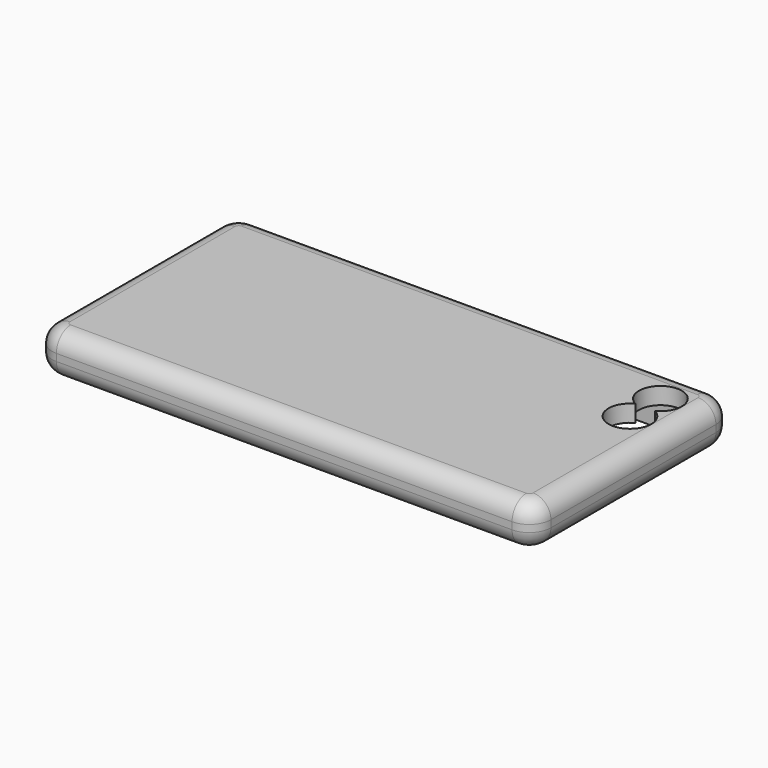
from build123d import *

# Parameters (mm, degrees)
F0_W         = 142.24
F0_H         = 71.12
F1_DEPTH     = 12.192
F3_T         = -4.826
F4_D         = 12.192
F5_R         = 6.1468
F6_T1_DEPTH  = 129.9464
F6_T3_DEPTH  = 58.8264
F6_T6_ANGLE  = 90
F6_T8_ANGLE  = 90
F6_T10_ANGLE = 90
F6_T12_ANGLE = 90
F7_R         = 5.08


# Not quite as in the source:
# - a fillet or chamfer that OpenCascade refuses, or shapes differently, is made with other operations: its cross-section is extruded or revolved along the edge and cut away or added
# - a feature names something its author has since deleted; it is built from what else it names


with BuildPart() as f1:
    # F0 (on Top) → F1 (new body)
    with BuildSketch(Plane.XY):
        Rectangle(F0_W, F0_H)
    extrude(amount=F1_DEPTH)

    # F3
    f3_openings = [f1.faces().sort_by_distance(p)[0] for p in [
        (0, 0, 0),
    ]]
    offset(amount=F3_T, openings=f3_openings)

    # F4 (through all)
    with Locations(Plane(origin=(0, 0, 0), x_dir=(1, 0, 0), z_dir=(0, 0, -1))):
        with Locations((59.7701932977, -12.9658412188), (59.7701932977, -23.8187816803)):
            Hole(F4_D / 2)

    # F5
    f5_edges = [f1.edges().sort_by_distance(p)[0] for p in [
        (66.294, -30.734, 3.683),
        (66.294, 30.734, 3.683),
        (-66.294, 30.734, 3.683),
        (-66.294, -30.734, 3.683),
        (-71.12, 35.56, 6.096),
        (-71.12, -35.56, 6.096),
        (71.12, -35.56, 6.096),
        (71.12, 35.56, 6.096),
    ]]
    fillet(f5_edges, radius=F5_R)

    # F6: fillet of radius 5.08 on 1 edges, made by hand

    # F6_s2 → F6_t1 (cut)
    with BuildSketch(Plane.YZ.offset(-64.9732)):
        with BuildLine():
            ThreePointArc((30.48, 0), (34.0721024484, 1.4878975516), (35.56, 5.08))
            Line((35.56, 5.08), (35.56, 0))
            Line((35.56, 0), (30.48, 0))
        make_face()
        with BuildLine():
            ThreePointArc((-35.56, 5.08), (-34.0721024484, 1.4878975516), (-30.48, 0))
            Line((-30.48, 0), (-35.56, 0))
            Line((-35.56, 0), (-35.56, 5.08))
        make_face()
    extrude(amount=F6_T1_DEPTH, mode=Mode.SUBTRACT)

    # F6_s4 → F6_t3 (cut)
    with BuildSketch(Plane.XZ.offset(-29.4132)):
        with BuildLine():
            ThreePointArc((-66.04, 0), (-69.6321024484, 1.4878975516), (-71.12, 5.08))
            Line((-71.12, 5.08), (-71.12, 0))
            Line((-71.12, 0), (-66.04, 0))
        make_face()
        with BuildLine():
            ThreePointArc((66.04, 0), (69.6321024484, 1.4878975516), (71.12, 5.08))
            Line((71.12, 5.08), (71.12, 0))
            Line((71.12, 0), (66.04, 0))
        make_face()
    extrude(amount=F6_T3_DEPTH, mode=Mode.SUBTRACT)

    # F6_s5 → F6_t6 (revolve, cut)
    with BuildSketch(Plane.XZ.offset(-29.4132)):
        with BuildLine():
            ThreePointArc((66.04, 0), (69.6321024484, 1.4878975516), (71.12, 5.08))
            Line((71.12, 5.08), (71.12, 0))
            Line((71.12, 0), (66.04, 0))
        make_face()
    revolve(axis=Axis((64.9732, 29.4132, 0), (0, 0, 1)), revolution_arc=F6_T6_ANGLE, mode=Mode.SUBTRACT)

    # F6_s7 → F6_t8 (revolve, cut)
    with BuildSketch(Plane.XZ.offset(-29.4132)):
        with BuildLine():
            ThreePointArc((-66.04, 0), (-69.6321024484, 1.4878975516), (-71.12, 5.08))
            Line((-71.12, 5.08), (-71.12, 0))
            Line((-71.12, 0), (-66.04, 0))
        make_face()
    revolve(axis=Axis((-64.9732, 29.4132, 0), (0, 0, -1)), revolution_arc=F6_T8_ANGLE, mode=Mode.SUBTRACT)

    # F6_s9 → F6_t10 (revolve, cut)
    with BuildSketch(Plane.YZ.offset(-64.9732)):
        with BuildLine():
            ThreePointArc((-30.48, 0), (-34.0721024484, 1.4878975516), (-35.56, 5.08))
            Line((-35.56, 5.08), (-35.56, 0))
            Line((-35.56, 0), (-30.48, 0))
        make_face()
    revolve(axis=Axis((-64.9732, -29.4132, 0), (0, 0, -1)), revolution_arc=F6_T10_ANGLE, mode=Mode.SUBTRACT)

    # F6_s11 → F6_t12 (revolve, cut)
    with BuildSketch(Plane.YZ.offset(64.9732)):
        with BuildLine():
            ThreePointArc((-30.48, 0), (-34.0721024484, 1.4878975516), (-35.56, 5.08))
            Line((-35.56, 5.08), (-35.56, 0))
            Line((-35.56, 0), (-30.48, 0))
        make_face()
    revolve(axis=Axis((64.9732, -29.4132, 0), (0, 0, 1)), revolution_arc=F6_T12_ANGLE, mode=Mode.SUBTRACT)

    # F7
    f7_edges = [f1.edges().sort_by_distance(p)[0] for p in [
        (0, 35.56, 12.192),
        (69.319644, -33.759644, 12.192),
        (0, -35.56, 12.192),
        (-69.319644, -33.759644, 12.192),
        (-71.12, 0, 12.192),
        (71.12, 0, 12.192),
        (-69.319644, 33.759644, 12.192),
        (69.319644, 33.759644, 12.192),
    ]]
    fillet(f7_edges, radius=F7_R)


solid = f1.part
